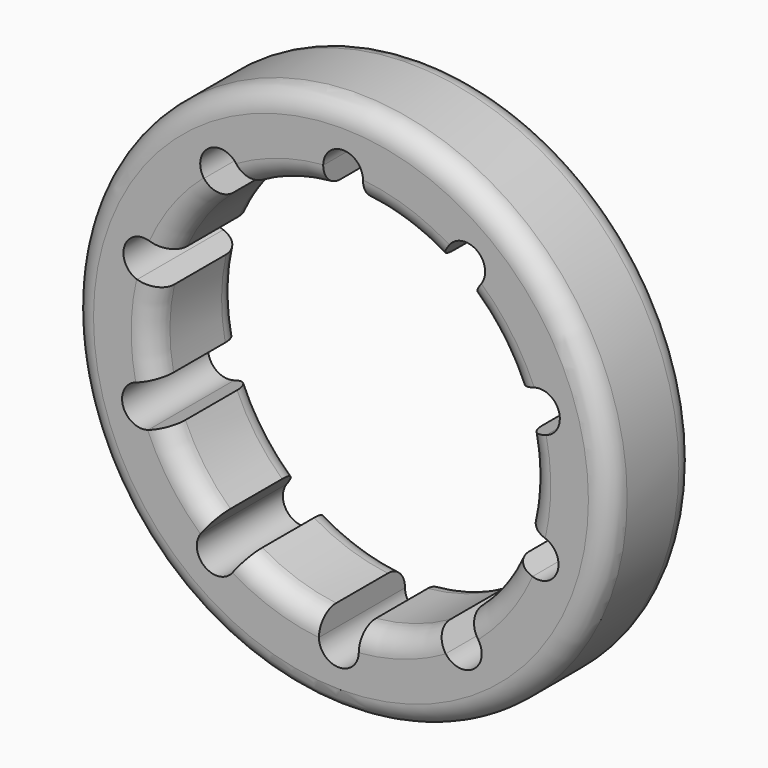
from build123d import *

# Parameters (mm, degrees)
F0_R     = 63.5
F0_R_2   = 44.45
F1_DEPTH = 25.4
F3_DEPTH = 25.4
F4_R     = 5.08
F5_R     = 5.08


with BuildPart() as f1:
    # F0 (on Front) → F1 (new body)
    with BuildSketch(Plane.XZ):
        Circle(F0_R)
        Circle(F0_R_2, mode=Mode.SUBTRACT)
    extrude(amount=F1_DEPTH)

    # F2 (on face) → F3 (cut)
    with BuildSketch(Plane.XZ.offset(25.4)):
        with BuildLine():
            ThreePointArc((-43.3835206407, 9.6784625235), (-42.1171755963, 14.2107712595), (-40.3787672252, 18.5838009398))
            Line((-40.3787672252, 18.5838009398), (-45.210134328, 20.1536072713))
            ThreePointArc((-45.210134328, 20.1536072713), (-51.1312197546, 17.1366635578), (-48.1142760411, 11.2155781311))
            Line((-48.1142760411, 11.2155781311), (-43.3835206407, 9.6784625235))
        make_face()
        with BuildLine():
            ThreePointArc((-29.409147938, 33.330234286), (-25.7206290425, 36.2526101358), (-21.7438247731, 38.7686546612))
            Line((-21.7438247731, 38.7686546612), (-24.7297738548, 42.8784609926))
            ThreePointArc((-24.7297738548, 42.8784609926), (-31.2933476119, 43.9180289486), (-32.3329155679, 37.3544551915))
            Line((-32.3329155679, 37.3544551915), (-29.409147938, 33.330234286))
        make_face()
        with BuildLine():
            Line((-4.2014803031, 49.2252), (-4.2014803031, 44.2509894043))
            ThreePointArc((-4.2014803031, 44.2509894043), (0.5003235936, 44.4471841212), (5.1965196969, 44.1452))
            Line((5.1965196969, 44.1452), (5.1965196969, 49.2252))
            ThreePointArc((5.1965196969, 49.2252), (0.4975196969, 53.9242), (-4.2014803031, 49.2252))
        make_face()
        with BuildLine():
            Line((25.5347776344, 42.2935915115), (22.6110100045, 38.269370606))
            ThreePointArc((22.6110100045, 38.269370606), (26.5301696223, 35.6644444765), (30.1519702659, 32.659779379))
            Line((30.1519702659, 32.659779379), (33.1379193475, 36.7695857104))
            ThreePointArc((33.1379193475, 36.7695857104), (32.0983513915, 43.3331594675), (25.5347776344, 42.2935915115))
        make_face()
        with BuildLine():
            Line((45.5176184107, 19.2072685719), (40.7868630103, 17.6701529642))
            ThreePointArc((40.7868630103, 17.6701529642), (42.4263925825, 13.2590992316), (43.5903930211, 8.6994331003))
            Line((43.5903930211, 8.6994331003), (48.4217601239, 10.2692394317))
            ThreePointArc((48.4217601239, 10.2692394317), (51.4387038374, 16.1903248584), (45.5176184107, 19.2072685719))
        make_face()
        with BuildLine():
            Line((48.1142760411, -11.2155781311), (43.3835206407, -9.6784625235))
            ThreePointArc((43.3835206407, -9.6784625235), (42.1171755963, -14.2107712595), (40.3787672252, -18.5838009398))
            Line((40.3787672252, -18.5838009398), (45.210134328, -20.1536072713))
            ThreePointArc((45.210134328, -20.1536072713), (51.1312197546, -17.1366635578), (48.1142760411, -11.2155781311))
        make_face()
        with BuildLine():
            Line((32.3329155679, -37.3544551915), (29.409147938, -33.330234286))
            ThreePointArc((29.409147938, -33.330234286), (25.7206290425, -36.2526101358), (21.7438247731, -38.7686546612))
            Line((21.7438247731, -38.7686546612), (24.7297738548, -42.8784609926))
            ThreePointArc((24.7297738548, -42.8784609926), (31.2933476119, -43.9180289486), (32.3329155679, -37.3544551915))
        make_face()
        with BuildLine():
            ThreePointArc((4.2014803031, -44.2509894043), (-0.5003235936, -44.4471841212), (-5.1965196969, -44.1452))
            Line((-5.1965196969, -44.1452), (-5.1965196969, -49.2252))
            ThreePointArc((-5.1965196969, -49.2252), (-0.4975196969, -53.9242), (4.2014803031, -49.2252))
            Line((4.2014803031, -49.2252), (4.2014803031, -44.2509894043))
        make_face()
        with BuildLine():
            ThreePointArc((-22.6110100045, -38.269370606), (-26.5301696223, -35.6644444765), (-30.1519702659, -32.659779379))
            Line((-30.1519702659, -32.659779379), (-33.1379193475, -36.7695857104))
            ThreePointArc((-33.1379193475, -36.7695857104), (-32.0983513915, -43.3331594675), (-25.5347776344, -42.2935915115))
            Line((-25.5347776344, -42.2935915115), (-22.6110100045, -38.269370606))
        make_face()
        with BuildLine():
            ThreePointArc((-40.7868630103, -17.6701529642), (-42.4263925825, -13.2590992316), (-43.5903930211, -8.6994331003))
            Line((-43.5903930211, -8.6994331003), (-48.4217601239, -10.2692394317))
            ThreePointArc((-48.4217601239, -10.2692394317), (-51.4387038374, -16.1903248584), (-45.5176184107, -19.2072685719))
            Line((-45.5176184107, -19.2072685719), (-40.7868630103, -17.6701529642))
        make_face()
    extrude(amount=-F3_DEPTH, mode=Mode.SUBTRACT)

    # F4
    f4_edges = [f1.edges().sort_by_distance(p)[0] for p in [
        (-35.664444, -25.4, 26.53017),
        (-13.259099, -25.4, 42.426393),
        (14.210771, -25.4, 42.117176),
        (36.25261, -25.4, 25.720629),
        (44.447184, -25.4, -0.500324),
        (35.664444, -25.4, -26.53017),
        (13.259099, -25.4, -42.426393),
        (-14.210771, -25.4, -42.117176),
        (-36.25261, -25.4, -25.720629),
        (-44.447184, -25.4, 0.500324),
        (-44.447184, 0, 0.500324),
        (-35.664444, 0, 26.53017),
        (-13.259099, 0, 42.426393),
        (14.210771, 0, 42.117176),
        (36.25261, 0, 25.720629),
        (-14.210771, 0, -42.117176),
        (-36.25261, 0, -25.720629),
        (13.259099, 0, -42.426393),
        (35.664444, 0, -26.53017),
        (44.447184, 0, -0.500324),
    ]]
    fillet(f4_edges, radius=F4_R)

    # F5
    f5_edges = [f1.edges().sort_by_distance(p)[0] for p in [
        (-63.5, -25.4, 0),
        (-63.5, 0, 0),
    ]]
    fillet(f5_edges, radius=F5_R)


solid = f1.part
